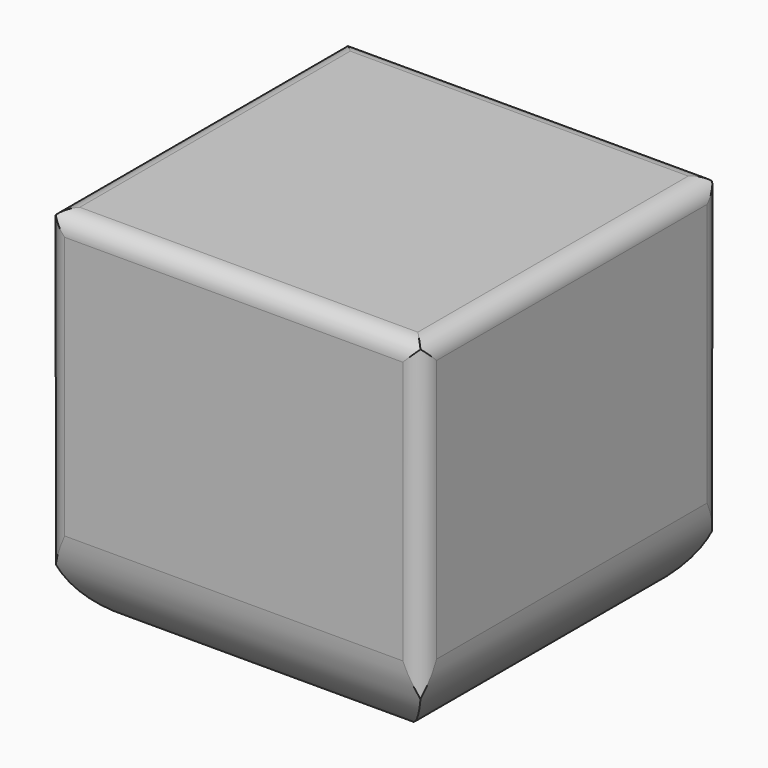
from build123d import *

# Parameters (mm, degrees)
F0_W        = 20
F0_H        = 20
F1_DEPTH    = 20
F2_R        = 5
F3_R        = 1
F4_T1_DEPTH = 20.75
F5_T1_DEPTH = 20.75


# Not quite as in the source:
# - a fillet or chamfer that OpenCascade refuses, or shapes differently, is made with other operations: its cross-section is extruded or revolved along the edge and cut away or added


with BuildPart() as f1:
    # F0 (on Front) → F1 (new body)
    with BuildSketch(Plane.XZ):
        with Locations((-5, 50)):
            Rectangle(F0_W, F0_H)
    extrude(amount=F1_DEPTH)

    # F2
    f2_edges = [f1.edges().sort_by_distance(p)[0] for p in [
        (-15, -10, 40),
        (5, -10, 40),
        (-5, 0, 40),
        (-5, -20, 40),
    ]]
    fillet(f2_edges, radius=F2_R)

    # F3
    f3_edges = [f1.edges().sort_by_distance(p)[0] for p in [
        (5, -10, 60),
        (-15, -10, 60),
        (-5, 0, 60),
        (-5, -20, 60),
    ]]
    fillet(f3_edges, radius=F3_R)

    # F4: fillet of radius 1 on 4 edges, made by hand

    # F4_s2 → F4_t1 (cut)
    with BuildSketch(Plane.XY.offset(40.75)):
        with BuildLine():
            ThreePointArc((4, 0), (4.7071067812, -0.2928932188), (5, -1))
            Line((5, -1), (5, 0))
            Line((5, 0), (4, 0))
        make_face()
        with BuildLine():
            ThreePointArc((4, -20), (4.7071067812, -19.7071067812), (5, -19))
            Line((5, -19), (5, -20))
            Line((5, -20), (4, -20))
        make_face()
    extrude(amount=F4_T1_DEPTH, mode=Mode.SUBTRACT)

    # F5: fillet of radius 1 on 4 edges, made by hand

    # F5_s2 → F5_t1 (cut)
    with BuildSketch(Plane.XY.offset(40.75)):
        with BuildLine():
            ThreePointArc((-15, -1), (-14.7071067812, -0.2928932188), (-14, 0))
            Line((-14, 0), (-15, 0))
            Line((-15, 0), (-15, -1))
        make_face()
        with BuildLine():
            ThreePointArc((-15, -19), (-14.7071067812, -19.7071067812), (-14, -20))
            Line((-14, -20), (-15, -20))
            Line((-15, -20), (-15, -19))
        make_face()
    extrude(amount=F5_T1_DEPTH, mode=Mode.SUBTRACT)


solid = f1.part
